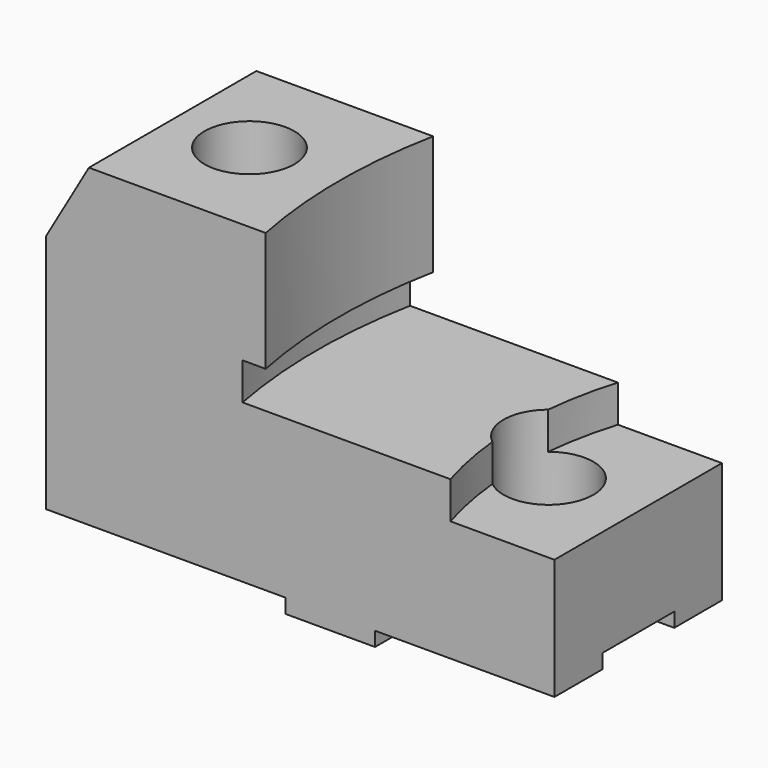
from build123d import *

# Parameters (mm, degrees)
F0_W                   = 107.95
F0_H                   = 69.85
F1_DEPTH               = 44.45
F2_W                   = 50.8254
F2_H                   = 3.048
F2_W_2                 = 38.1
F3_DEPTH               = 66.64201
F3_DEPTH_BACK          = 161
F4_W                   = 19.1008
F4_H                   = 3.048
F4_H_2                 = 17.1056788669
F5_DEPTH               = 107.951
F7_DEPTH               = 33.274
F9_W                   = 18.9599941809
F9_H                   = 7.874
F11_W                  = 28.8704986477
F11_H                  = 14.4021337534
F12_ANGLE_BACK         = 30
F12_ANGLE              = 60
F15_D                  = 12.7
F15_CBORE_D            = 19.05
F15_CBORE_DEPTH        = 20.574
F15_ON_F14_D           = 12.7
F15_ON_F14_START       = 7.874
F15_ON_F14_CBORE_D     = 19.05
F15_ON_F14_CBORE_DEPTH = 20.574


# Not quite as in the source:
# - an extrude ends at something that could not be found from the text; its depth is read off the source's solid
# - a length typed as a fraction of an inch, garbled in the dataset ("3 / 203.2 mm" for 3/8 in), is restored


with BuildPart() as f1:
    # F0 (on Front) → F1 (new body)
    with BuildSketch(Plane.XZ):
        with Locations((0.967470929, 9.7001004595)):
            Rectangle(F0_W, F0_H)
    extrude(amount=F1_DEPTH)

    # F2 (on face) → F3 (cut, two sides)
    with BuildSketch(Plane.XZ.offset(44.45)) as f3_sk:
        with Locations((-27.594829071, -23.7008995405)):
            Rectangle(F2_W, F2_H)
        with Locations((35.892470929, -23.7008995405)):
            Rectangle(F2_W_2, F2_H)
        Polygon((-53.007529071, 44.6251004595), (-43.9154170318, 44.6251004595), (-53.007529071, 49.8744337929), (-64.4665259088, 30.026869066), (-53.007529071, 28.8771004595), align=None)
        Polygon((-53.007529071, 28.8771004595), (-43.9154170318, 44.6251004595), (-53.007529071, 44.6251004595), align=None)
    extrude(amount=-F3_DEPTH, mode=Mode.SUBTRACT)
    extrude(f3_sk.sketch, amount=F3_DEPTH_BACK, mode=Mode.SUBTRACT)

    # F4 (on face) → F5 (cut, through all)
    with BuildSketch(Plane.YZ.offset(54.942470929)):
        with Locations((-22.1996, -20.6528995405)):
            Rectangle(F4_W, F4_H)
        with Locations((-22.1996, -30.7297389739)):
            Rectangle(F4_W, F4_H_2)
    extrude(amount=-F5_DEPTH, mode=Mode.SUBTRACT)

    # F6 (on face) → F7 (cut)
    with BuildSketch(Plane.XY.offset(44.6251004595)):
        with BuildLine():
            Line((84.230268681, 4.7385622747), (-0.8366582079, 19.0712375092))
            ThreePointArc((-0.8366582079, 19.0712375092), (-8.5367916359, -24.4021880093), (0.8136185269, -67.5507755982))
            Line((0.8136185269, -67.5507755982), (81.3293292463, -56.9063611329))
            Line((81.3293292463, -56.9063611329), (105.742470929, -22.225))
            Line((105.742470929, -22.225), (84.230268681, 4.7385622747))
        make_face()
    extrude(amount=-F7_DEPTH, mode=Mode.SUBTRACT)

    # F9 (on offset) → F10 (revolve, cut)
    with BuildSketch(Plane.XZ.offset(22.225)):
        with Locations((-3.9035319805, 15.2881004595)):
            Rectangle(F9_W, F9_H)
    revolve(axis=Axis((105.742470929, -22.225, 44.6251004595), (0, 0, 1)), mode=Mode.SUBTRACT)

    # F11 (on offset) → F12 (revolve, cut)
    with BuildSketch(Plane.XZ.offset(22.225), mode=Mode.PRIVATE) as f12_sk:
        with Locations((43.9777202529, 10.6781673362)):
            Rectangle(F11_W, F11_H)
    revolve(f12_sk.sketch.rotate(Axis((105.742470929, -22.225, 44.6251004595), (0, 0, -1)), -F12_ANGLE_BACK), axis=Axis((105.742470929, -22.225, 44.6251004595), (0, 0, -1)), revolution_arc=F12_ANGLE, mode=Mode.SUBTRACT)

    # F15 (through all)
    with Locations(Plane.XY.offset(44.6251004595)):
        with Locations((-27.607529071, -22.225)):
            CounterBoreHole(F15_D / 2, F15_CBORE_D / 2, F15_CBORE_DEPTH)

    # F15 on F14 (through all)
    # its depths count from where the whole tool has entered the part; down to there all is cleared
    with Locations(Plane.XY.offset(11.3511004595).offset(-F15_ON_F14_START)):
        with Locations((35.892470929, -22.225)):
            CounterBoreHole(F15_ON_F14_D / 2, F15_ON_F14_CBORE_D / 2, F15_ON_F14_CBORE_DEPTH)


solid = f1.part
